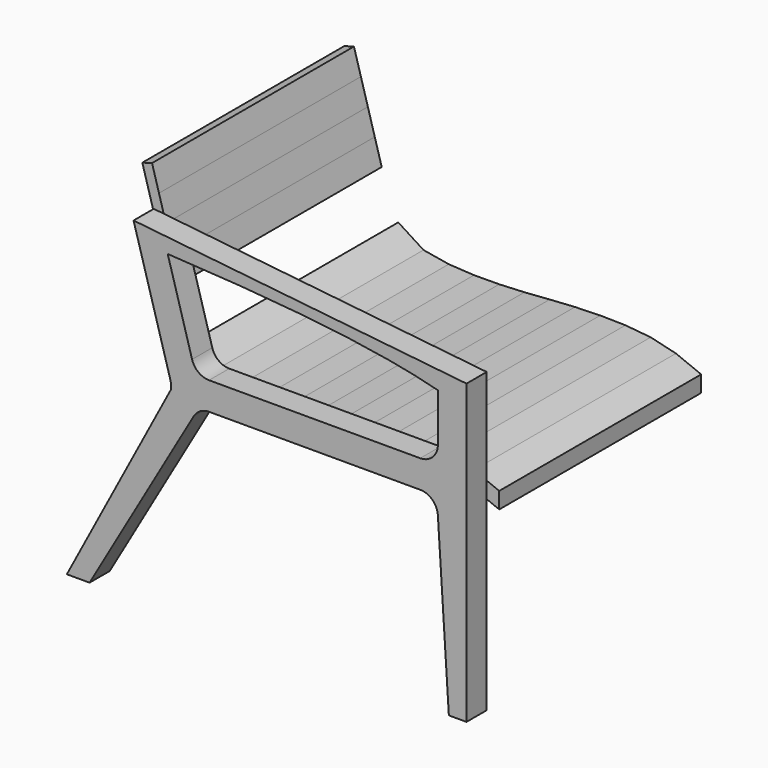
from build123d import *

# Parameters (mm, degrees)
F2_DEPTH = 500
F3_DEPTH = 50


with BuildPart() as f2:
    # F1 (on Front) → F2 (new body)
    with BuildSketch(Plane.XZ):
        Polygon((-313.022685147, 308.6738246905), (-332.2518732106, 303.1748860281), (-318.5045265546, 255.101915869), (-299.275338491, 260.6008545314), align=None)
        Polygon((-299.275338491, 260.6008545314), (-318.5045265546, 255.101915869), (-304.7571798986, 207.0289457099), (-285.5279918349, 212.5278843723), align=None)
        Polygon((-285.5279918349, 212.5278843723), (-304.7571798986, 207.0289457099), (-291.0098332425, 158.9559755508), (-271.7806451789, 164.4549142132), align=None)
        Polygon((-271.7806451789, 164.4549142132), (-291.0098332425, 158.9559755508), (-277.2624865865, 110.8830053917), (-258.0332985228, 116.3819440541), align=None)
    extrude(amount=-F2_DEPTH)


with BuildPart() as f2b:
    # F1 (on Front) → F2, piece 2 (new body)
    with BuildSketch(Plane.XZ):
        Polygon((374.7528376444, -39.4042041541), (324.7528376444, -19.1975054732), (324.7528376444, -51.5547587832), (374.7528376444, -71.7614574641), align=None)
        Polygon((324.7528376444, -51.5547587832), (324.7528376444, -19.1975054732), (274.7528376444, -7.2214900208), (274.7528376444, -38.0700391051), align=None)
        Polygon((274.7528376444, -38.0700391051), (274.7528376444, -7.2214900208), (224.7528376444, -2.5200431725), (224.7528376444, -32.6523729345), align=None)
        Polygon((224.7528376444, -32.6523729345), (224.7528376444, -2.5200431725), (174.7528376444, -1.656131361), (174.7528376444, -31.670252785), align=None)
        Polygon((174.7528376444, -31.670252785), (174.7528376444, -1.656131361), (124.7528376444, -3.1904470413), (124.7528376444, -33.25025125), align=None)
        Polygon((124.7528376444, -33.25025125), (124.7528376444, -3.1904470413), (74.7528376444, -6.3491339475), (74.7528376444, -36.2796506691), align=None)
        Polygon((74.7528376444, -36.2796506691), (74.7528376444, -6.3491339475), (24.7528376444, -10.0282630796), (24.7528376444, -40.061218899), align=None)
        Polygon((24.7528376444, -40.061218899), (24.7528376444, -10.0282630796), (-25.2471623556, -12.3725440927), (-25.2471623556, -42.3731500731), align=None)
        with BuildLine():
            Line((-25.2471623556, -42.3731500731), (-25.2471623556, -12.3725440927))
            Line((-25.2471623556, -12.3725440927), (-60.3584851816, -12.5957126798))
            add(Edge.make_bspline(
                [(-60.3584851816, -12.5957126798), (-56.9180854904, -21.5284331632), (-55.115206892, -31.8869926762), (-53.7958883398, -42.5546066042)],
                knots=[0.8239164259, 0.8239164259, 0.8239164259, 0.8239164259, 0.9454560047, 0.9454560047, 0.9454560047, 0.9454560047], degree=3))
            Line((-53.7958883398, -42.5546066042), (-25.2471623556, -42.3731500731))
        make_face()
        with BuildLine():
            add(Edge.make_bspline(
                [(-60.3584851816, -12.5957126798), (-56.9180854904, -21.5284331632), (-55.115206892, -31.8869926762), (-53.7958883398, -42.5546066042)],
                knots=[0.8239164259, 0.8239164259, 0.8239164259, 0.8239164259, 0.9454560047, 0.9454560047, 0.9454560047, 0.9454560047], degree=3))
            Line((-60.3584851816, -12.5957126798), (-75.2471623556, -12.6903455441))
            Line((-75.2471623556, -12.6903455441), (-75.2471623556, -42.6909515245))
            Line((-75.2471623556, -42.6909515245), (-53.7958883398, -42.5546066042))
        make_face()
        with BuildLine():
            Line((-175.2471623556, -1.3737931919), (-185.149231833, 4.9516693116))
            add(Edge.make_bspline(
                [(-225.2471623556, 3.6267801279), (-218.5699288591, 0.1086035939), (-203.4752736384, 1.8377965797), (-185.149231833, 4.9516693116)],
                knots=[0.2038986096, 0.2038986096, 0.2038986096, 0.2038986096, 0.368291831, 0.368291831, 0.368291831, 0.368291831], degree=3))
            Line((-225.2471623556, 3.6267801279), (-225.2471623556, -4.6656222887))
            Line((-225.2471623556, -4.6656222887), (-175.2471623556, -31.8025045694))
            Line((-175.2471623556, -31.8025045694), (-175.2471623556, -1.3737931919))
        make_face()
        with BuildLine():
            add(Edge.make_bspline(
                [(-225.2471623556, 3.6267801279), (-218.5699288591, 0.1086035939), (-203.4752736384, 1.8377965797), (-185.149231833, 4.9516693116)],
                knots=[0.2038986096, 0.2038986096, 0.2038986096, 0.2038986096, 0.368291831, 0.368291831, 0.368291831, 0.368291831], degree=3))
            Line((-185.149231833, 4.9516693116), (-225.2471623556, 30.5663104296))
            Line((-225.2471623556, 30.5663104296), (-225.2471623556, 3.6267801279))
        make_face()
        Polygon((-75.2471623556, -42.6909515245), (-75.2471623556, -12.6903455441), (-125.2471623556, -9.8568606564), (-125.2471623556, -39.9049938626), align=None)
        Polygon((-125.2471623556, -9.8568606564), (-175.2471623556, -1.3737931919), (-175.2471623556, -31.8025045694), (-125.2471623556, -39.9049938626), align=None)
    extrude(amount=-F2_DEPTH)


with BuildPart() as f2c:
    # F1 (on Front) → F2, piece 3 (new body)
    with BuildSketch(Plane.XZ):
        Polygon((-231.5898423556, -1.4372480625), (-231.5898423556, -1.4286871489), (-231.5917925852, -1.4274861968), align=None)
    extrude(amount=-F2_DEPTH)


with BuildPart() as f3:
    # F0 (on Front) → F3 (new body)
    with BuildSketch(Plane.XZ):
        with BuildLine():
            ThreePointArc((-160.0633602421, -55), (-166.7365377228, -27.5), (-160.0633602421, 0))
            ThreePointArc((-160.0633602421, 0), (-181.1268860524, 7.0477571483), (-193.7075195999, 25.3526925464))
            Line((-193.7075195999, 25.3526925464), (-241.9597391517, 193.6281799587))
            Line((-241.9597391517, 193.6281799587), (-309.6056596926, 230))
            Line((-309.6056596926, 230), (-237.122271712, -22.7796141821))
            ThreePointArc((-237.122271712, -22.7796141821), (-236.0889018962, -27.0990222261), (-235.4429058376, -31.4930896038))
            ThreePointArc((-235.4429058376, -31.4930896038), (-235.1893804809, -35.9271468791), (-235.3303261555, -40.3662090936))
            Line((-235.3303261555, -40.3662090936), (-441.7769706098, -430))
            Line((-441.7769706098, -430), (-396.7769706098, -430))
            Line((-396.7769706098, -430), (-190.3742493745, -72.5))
            ThreePointArc((-190.3742493745, -72.5), (-177.5633602421, -59.6891108675), (-160.0633602421, -55))
        make_face()
        with BuildLine():
            Line((258.2606234636, 0), (-160.0633602421, 0))
            ThreePointArc((-160.0633602421, 0), (-166.7365377228, -27.5), (-160.0633602421, -55))
            Line((-160.0633602421, -55), (258.2606234636, -55))
            ThreePointArc((258.2606234636, -55), (264.9338009444, -27.5), (258.2606234636, 0))
        make_face()
        with BuildLine():
            ThreePointArc((293.2606234636, 35), (283.0093608052, 10.2512626585), (258.2606234636, 0))
            ThreePointArc((258.2606234636, 0), (264.9338009444, -27.5), (258.2606234636, -55))
            ThreePointArc((258.2606234636, -55), (282.2117573173, -64.4785739598), (293.1901715336, -87.7803893072))
            Line((293.1901715336, -87.7803893072), (314.9366397579, -430))
            Line((314.9366397579, -430), (348.9601495671, -430))
            Line((348.9601495671, -430), (349.7293803363, -430))
            Line((349.7293803363, -430), (349.9366397579, -430))
            Line((349.9366397579, -430), (349.9366397579, 112.6860928485))
            add(Edge.make_bspline(
                [(293.2606234636, 130), (313.447396449, 124.6358037529), (332.2966423185, 118.8506913972), (349.9366397579, 112.6860928485)],
                knots=[0.6174610646, 0.6174610646, 0.6174610646, 0.6174610646, 0.7111631147, 0.7111631147, 0.7111631147, 0.7111631147], degree=3))
            Line((293.2606234636, 130), (293.2606234636, 35))
        make_face()
        with BuildLine():
            Line((-309.6056596926, 230), (-241.9597391517, 193.6281799587))
            add(Edge.make_bspline(
                [(-241.9597391517, 193.6281799587), (-30.8653650886, 182.4185598631), (160.2374256996, 165.3480241113), (293.2606234636, 130)],
                knots=[0, 0, 0, 0, 0.6174610646, 0.6174610646, 0.6174610646, 0.6174610646], degree=3))
            Line((293.2606234636, 130), (349.9366397579, 160))
            Line((349.9366397579, 160), (-309.6056596926, 230))
        make_face()
        with BuildLine():
            Line((349.9366397579, 160), (293.2606234636, 130))
            add(Edge.make_bspline(
                [(293.2606234636, 130), (313.447396449, 124.6358037529), (332.2966423185, 118.8506913972), (349.9366397579, 112.6860928485)],
                knots=[0.6174610646, 0.6174610646, 0.6174610646, 0.6174610646, 0.7111631147, 0.7111631147, 0.7111631147, 0.7111631147], degree=3))
            Line((349.9366397579, 112.6860928485), (349.9366397579, 160))
        make_face()
    extrude(amount=F3_DEPTH)


solid = Compound([f2.part, f2b.part, f2c.part, f3.part])
